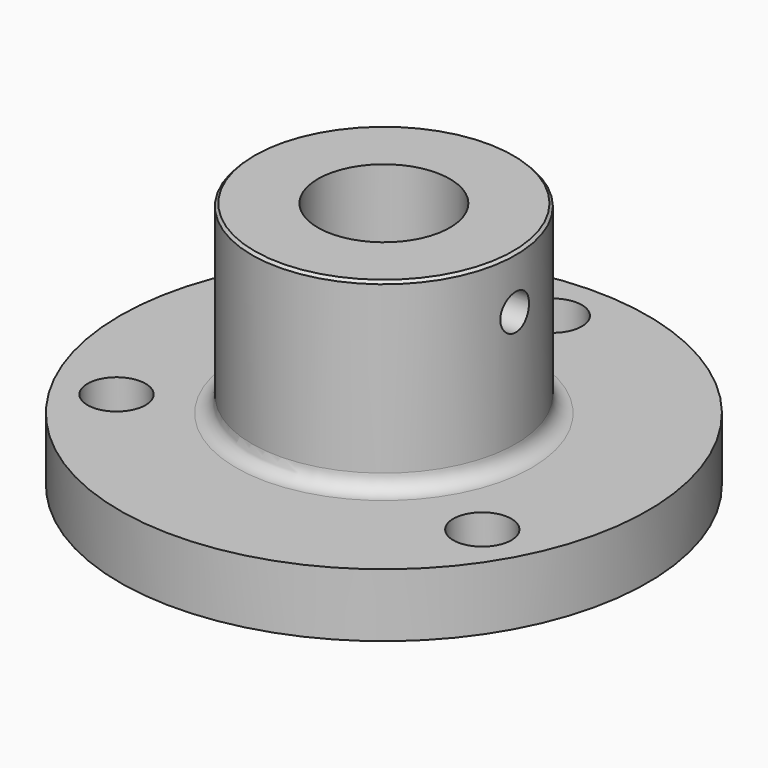
from build123d import *

# Parameters (mm, degrees)
F2_R            = 3
F4_D            = 6.8
F4_DEPTH        = 50.001
F5_R            = 5.5
F6_DEPTH        = 15.0010001
F6_COPIES_COUNT = 3
F7_SIZE         = 0.5


# Not quite as in the source:
# - a pattern or mirror of a feature is missing from the dataset's text; its kind, count and spacing are read off the source's solid


with BuildPart() as f1:
    # F0 (on Front) → F1 (revolve)
    with BuildSketch(Plane.XZ):
        Polygon((-20, 0), (-12.5, 0), (-12.5, 50), (-25, 50), (-25, 15), (-50, 15), (-50, 3), (-20, 3), align=None)
    revolve(axis=Axis((0, 0, 33.7237479181), (0, 0, 1)))

    # F2
    f2_edges = [f1.edges().sort_by_distance(p)[0] for p in [
        (25, 0, 15),
    ]]
    fillet(f2_edges, radius=F2_R)

    # F4 (through all, one way)
    with BuildSketch(Plane(origin=(0, 0, 0), x_dir=(0, 1, 0), z_dir=(-1, 0, 0))):
        with Locations((0, -40)):
            Circle(F4_D / 2)
    extrude(amount=-F4_DEPTH, mode=Mode.SUBTRACT)

    # F5 (on face) → F6 (cut, through all)
    with BuildSketch(Plane.XY.offset(15)):
        with Locations((0, 40)):
            Circle(F5_R)
    f6 = extrude(amount=-F6_DEPTH, mode=Mode.SUBTRACT)

    # F6_copies: F6 ×3 about axis
    f6_copies_axis = Axis((0, 0, 0), (0, 0, 1))
    for i in range(1, F6_COPIES_COUNT):
        add(f6.rotate(f6_copies_axis, i * 360 / F6_COPIES_COUNT), mode=Mode.SUBTRACT)

    # F7
    f7_edges = [f1.edges().sort_by_distance(p)[0] for p in [
        (25, 0, 50),
    ]]
    chamfer(f7_edges, length=F7_SIZE)


solid = f1.part
